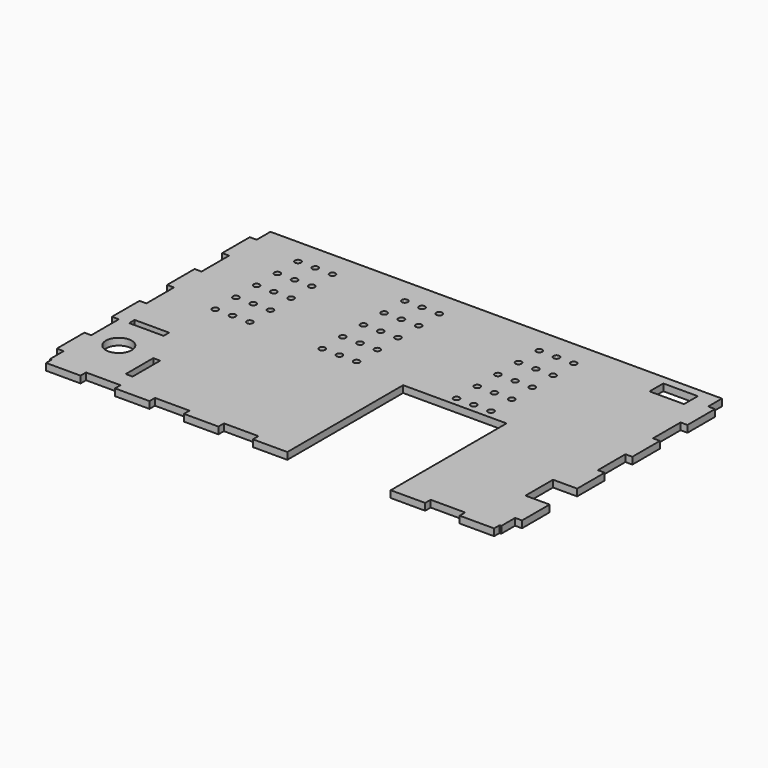
from build123d import *

# Parameters (mm, degrees)
F0_R     = 7.5
F0_W     = 4
F0_H     = 20
F0_W_2   = 20
F0_H_2   = 4
F0_R_2   = 1.75
F0_H_3   = 10
F1_DEPTH = 4


# Not quite as in the source:
# - ends of sketch curves that miss each other by under 0.0002 mm in the source are joined


with BuildPart() as f1:
    # F0 (on Top) → F1 (new body)
    with BuildSketch(Plane.XY):
        Polygon((-21.444316276, -128.1282028952), (-1.444316276, -128.1282028952), (-1.444316276, -124.1282028952), (-1.444316276, -44.1282028952), (58.555683724, -44.1282028952), (58.555683724, -124.1282028952), (58.555683724, -128.1282028952), (78.555683724, -128.1282028952), (78.555683724, -124.1282028952), (98.555683724, -124.1282028952), (98.555683724, -128.1282028952), (118.555683724, -128.1282028952), (118.555683724, -124.1282028952), (119.555683724, -124.1282028952), (119.555683724, -114.1282028952), (123.555683724, -114.1282028952), (123.5556837228, -94.1282028952), (119.5556837228, -94.1282028952), (109.5556834554, -94.1282028952), (109.5556834554, -74.1282028952), (119.5556834554, -74.1282028952), (123.555683724, -74.1282028952), (123.5556837228, -54.1282028952), (119.5556837228, -54.1282028952), (119.5556837242, -34.1282028952), (123.555683724, -34.1282028952), (123.5556837228, -14.1282028952), (119.5556837228, -14.1282028952), (119.5556837242, 5.8717971048), (123.555683724, 5.8717971048), (123.5556837228, 25.8717971048), (119.5556837228, 25.8717971048), (119.555683724, 35.8717971048), (-142.444316276, 35.8717971048), (-142.4443162747, 25.8717971048), (-146.4443162747, 25.8717971048), (-146.444316276, 5.8717971048), (-142.444316276, 5.8717971048), (-142.4443162747, -14.1282028952), (-146.4443162747, -14.1282028952), (-146.444316276, -34.1282028952), (-142.444316276, -34.1282028952), (-142.4443162747, -54.1282028952), (-146.4443162747, -54.1282028952), (-146.444316276, -74.1282028952), (-142.444316276, -74.1282028952), (-142.4443162747, -94.1282028952), (-146.4443162747, -94.1282028952), (-146.444316276, -114.1282028952), (-142.444316276, -114.1282028952), (-142.444316276, -124.1282028952), (-141.444316276, -124.1282028952), (-141.444316276, -128.1282028952), (-121.444316276, -128.1282028952), (-121.444316276, -124.1282028952), (-101.444316276, -124.1282028952), (-101.444316276, -128.1282028952), (-81.444316276, -128.1282028952), (-81.444316276, -124.1282028952), (-61.444316276, -124.1282028952), (-61.444316276, -128.1282028952), (-41.444316276, -128.1282028952), (-41.444316276, -124.1282028952), (-21.444316276, -124.1282028952), align=None)
        with Locations((-126.4443162747, -94.1282028952)):
            Circle(F0_R, mode=Mode.SUBTRACT)
        with Locations((-104.4443162747, -104.1282028952)):
            Rectangle(F0_W, F0_H, mode=Mode.SUBTRACT)
        with Locations((-126.4443162747, -72.1282028948)):
            Rectangle(F0_W_2, F0_H_2, mode=Mode.SUBTRACT)
        with Locations((-114.444316276, -39.1282028952)):
            Circle(F0_R_2, mode=Mode.SUBTRACT)
        with Locations((-104.444316276, -39.1282028952)):
            Circle(F0_R_2, mode=Mode.SUBTRACT)
        with Locations((-94.444316276, -39.1282028952)):
            Circle(F0_R_2, mode=Mode.SUBTRACT)
        with Locations((-114.444316276, -24.1282028952)):
            Circle(F0_R_2, mode=Mode.SUBTRACT)
        with Locations((-114.444316276, -9.1282028952)):
            Circle(F0_R_2, mode=Mode.SUBTRACT)
        with Locations((-104.444316276, -24.1282028952)):
            Circle(F0_R_2, mode=Mode.SUBTRACT)
        with Locations((-94.444316276, -24.1282028952)):
            Circle(F0_R_2, mode=Mode.SUBTRACT)
        with Locations((-104.444316276, -9.1282028952)):
            Circle(F0_R_2, mode=Mode.SUBTRACT)
        with Locations((-94.444316276, -9.1282028952)):
            Circle(F0_R_2, mode=Mode.SUBTRACT)
        with Locations((-52.444316276, -39.1282028952)):
            Circle(F0_R_2, mode=Mode.SUBTRACT)
        with Locations((-42.444316276, -39.1282028952)):
            Circle(F0_R_2, mode=Mode.SUBTRACT)
        with Locations((-32.444316276, -39.1282028952)):
            Circle(F0_R_2, mode=Mode.SUBTRACT)
        with Locations((-52.444316276, -24.1282028952)):
            Circle(F0_R_2, mode=Mode.SUBTRACT)
        with Locations((-52.444316276, -9.1282028952)):
            Circle(F0_R_2, mode=Mode.SUBTRACT)
        with Locations((-42.444316276, -24.1282028952)):
            Circle(F0_R_2, mode=Mode.SUBTRACT)
        with Locations((-32.444316276, -24.1282028952)):
            Circle(F0_R_2, mode=Mode.SUBTRACT)
        with Locations((-42.444316276, -9.1282028952)):
            Circle(F0_R_2, mode=Mode.SUBTRACT)
        with Locations((-32.444316276, -9.1282028952)):
            Circle(F0_R_2, mode=Mode.SUBTRACT)
        with Locations((-114.444316276, 5.8717971048)):
            Circle(F0_R_2, mode=Mode.SUBTRACT)
        with Locations((-104.444316276, 5.8717971048)):
            Circle(F0_R_2, mode=Mode.SUBTRACT)
        with Locations((-94.444316276, 5.8717971048)):
            Circle(F0_R_2, mode=Mode.SUBTRACT)
        with Locations((-114.444316276, 20.8717971048)):
            Circle(F0_R_2, mode=Mode.SUBTRACT)
        with Locations((-104.444316276, 20.8717971048)):
            Circle(F0_R_2, mode=Mode.SUBTRACT)
        with Locations((-94.444316276, 20.8717971048)):
            Circle(F0_R_2, mode=Mode.SUBTRACT)
        with Locations((-52.444316276, 5.8717971048)):
            Circle(F0_R_2, mode=Mode.SUBTRACT)
        with Locations((-42.444316276, 5.8717971048)):
            Circle(F0_R_2, mode=Mode.SUBTRACT)
        with Locations((-32.444316276, 5.8717971048)):
            Circle(F0_R_2, mode=Mode.SUBTRACT)
        with Locations((-52.444316276, 20.8717971048)):
            Circle(F0_R_2, mode=Mode.SUBTRACT)
        with Locations((-42.444316276, 20.8717971048)):
            Circle(F0_R_2, mode=Mode.SUBTRACT)
        with Locations((-32.444316276, 20.8717971048)):
            Circle(F0_R_2, mode=Mode.SUBTRACT)
        with Locations((25.555683724, -39.1282028952)):
            Circle(F0_R_2, mode=Mode.SUBTRACT)
        with Locations((35.555683724, -39.1282028952)):
            Circle(F0_R_2, mode=Mode.SUBTRACT)
        with Locations((45.555683724, -39.1282028952)):
            Circle(F0_R_2, mode=Mode.SUBTRACT)
        with Locations((25.555683724, -24.1282028952)):
            Circle(F0_R_2, mode=Mode.SUBTRACT)
        with Locations((35.555683724, -24.1282028952)):
            Circle(F0_R_2, mode=Mode.SUBTRACT)
        with Locations((45.555683724, -24.1282028952)):
            Circle(F0_R_2, mode=Mode.SUBTRACT)
        with Locations((25.555683724, -9.1282028952)):
            Circle(F0_R_2, mode=Mode.SUBTRACT)
        with Locations((35.555683724, -9.1282028952)):
            Circle(F0_R_2, mode=Mode.SUBTRACT)
        with Locations((45.555683724, -9.1282028952)):
            Circle(F0_R_2, mode=Mode.SUBTRACT)
        with Locations((25.555683724, 5.8717971048)):
            Circle(F0_R_2, mode=Mode.SUBTRACT)
        with Locations((35.555683724, 5.8717971048)):
            Circle(F0_R_2, mode=Mode.SUBTRACT)
        with Locations((45.555683724, 5.8717971048)):
            Circle(F0_R_2, mode=Mode.SUBTRACT)
        with Locations((25.555683724, 20.8717971048)):
            Circle(F0_R_2, mode=Mode.SUBTRACT)
        with Locations((35.555683724, 20.8717971048)):
            Circle(F0_R_2, mode=Mode.SUBTRACT)
        with Locations((45.555683724, 20.8717971048)):
            Circle(F0_R_2, mode=Mode.SUBTRACT)
        with Locations((99.555683724, 25.8717971048)):
            Rectangle(F0_W_2, F0_H_3, mode=Mode.SUBTRACT)
    extrude(amount=F1_DEPTH)


solid = f1.part
